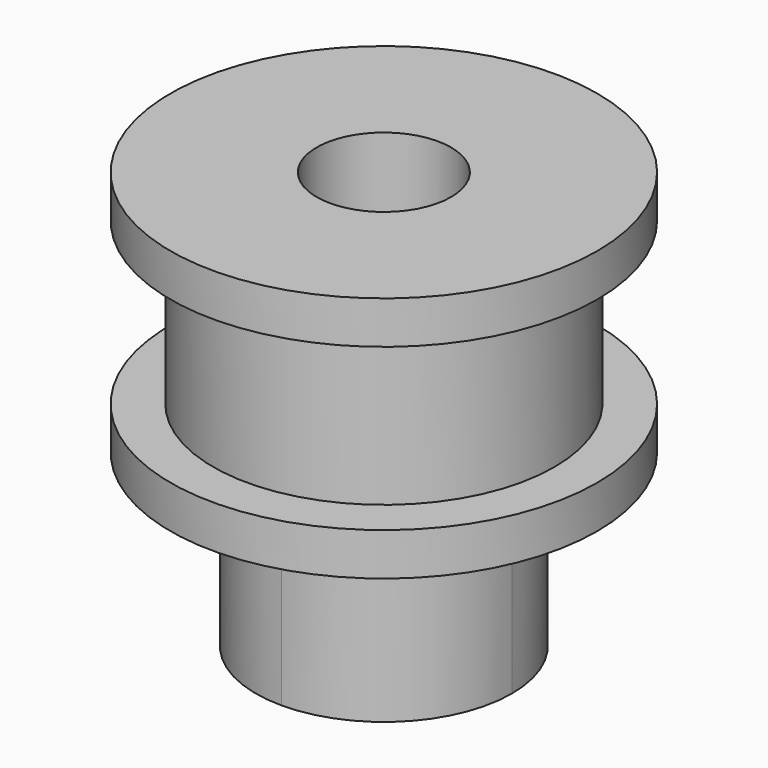
from build123d import *

# Parameters (mm, degrees)
F0_R         = 6.35
F1_DEPTH     = 6
F2_R         = 7.9375
F3_DEPTH     = 1.5875
F4_R         = 7.9375
F5_DEPTH     = 1.5875
F6_W         = 9.525
F6_H         = 9.525
F7_DEPTH     = 6.35
F8_R         = 2.5
F9_DEPTH     = 15.525
F11_REACH    = 16.5631366107
F12_T1_DEPTH = 18.25625


# Not quite as in the source:
# - a fillet or chamfer that OpenCascade refuses, or shapes differently, is made with other operations: its cross-section is extruded or revolved along the edge and cut away or added


with BuildPart() as f1:
    # F0 (on Top) → F1 (new body)
    with BuildSketch(Plane.XY):
        Circle(F0_R)
    extrude(amount=F1_DEPTH)

    # F2 (on face) → F3 (join)
    with BuildSketch(Plane.XY.offset(6)):
        Circle(F2_R)
    extrude(amount=F3_DEPTH)

    # F4 (on face) → F5 (join)
    with BuildSketch(Plane(origin=(0, 0, 0), x_dir=(1, 0, 0), z_dir=(0, 0, -1))):
        Circle(F4_R)
    extrude(amount=F5_DEPTH)

    # F6 (on face) → F7 (join)
    with BuildSketch(Plane(origin=(0, 0, -1.5875), x_dir=(1, 0, 0), z_dir=(0, 0, -1))):
        Rectangle(F6_W, F6_H)
    extrude(amount=F7_DEPTH)

    # F8 (on face) → F9 (cut, through all)
    with BuildSketch(Plane(origin=(0, 0, -7.9375), x_dir=(1, 0, 0), z_dir=(0, 0, -1))):
        Circle(F8_R)
    extrude(amount=-F9_DEPTH, mode=Mode.SUBTRACT)

    f11_end = f1.faces().sort_by_distance((-2.5, 0, -0.175))[0]
    # F10 (on face) → F11 (cut, up to a face of the model that its end follows)
    with BuildSketch(Plane(origin=(-4.7625, 0, 0), x_dir=(0, -1, 0), z_dir=(-1, 0, 0))):
        with BuildLine():
            ThreePointArc((0, -3.0353), (-1.7272, -4.7625), (0, -6.4897))
            Line((0, -6.4897), (0, -3.0353))
        make_face()
        with BuildLine():
            Line((0, -3.0353), (0, -6.4897))
            ThreePointArc((0, -6.4897), (1.2213148325, -5.9838148325), (1.7272, -4.7625))
            ThreePointArc((1.7272, -4.7625), (1.2213148325, -3.5411851675), (0, -3.0353))
        make_face()
    f11_long = extrude(amount=-F11_REACH, mode=Mode.PRIVATE)
    add(split(f11_long, bisect_by=f11_end, keep=Keep.ALL, mode=Mode.PRIVATE).solids().sort_by_distance((-4.7625, 0, -4.7625))[0], mode=Mode.SUBTRACT)

    # F12: fillet of radius 4.7625 on 4 edges, made by hand

    # F12_s2 → F12_t1 (cut)
    with BuildSketch(Plane.XY.offset(-19.84375)):
        with BuildLine():
            ThreePointArc((-4.7625, 0), (-3.3675960454, -3.3675960454), (0, -4.7625))
            Line((0, -4.7625), (-4.7625, -4.7625))
            Line((-4.7625, -4.7625), (-4.7625, 0))
        make_face()
        with BuildLine():
            ThreePointArc((-4.7625, 0), (-3.3675960454, 3.3675960454), (0, 4.7625))
            Line((0, 4.7625), (-4.7625, 4.7625))
            Line((-4.7625, 4.7625), (-4.7625, 0))
        make_face()
        with BuildLine():
            ThreePointArc((0, 4.7625), (3.3675960454, 3.3675960454), (4.7625, 0))
            Line((4.7625, 0), (4.7625, 4.7625))
            Line((4.7625, 4.7625), (0, 4.7625))
        make_face()
        with BuildLine():
            ThreePointArc((4.7625, 0), (3.3675960454, -3.3675960454), (0, -4.7625))
            Line((0, -4.7625), (4.7625, -4.7625))
            Line((4.7625, -4.7625), (4.7625, 0))
        make_face()
    extrude(amount=F12_T1_DEPTH, mode=Mode.SUBTRACT)


solid = f1.part
